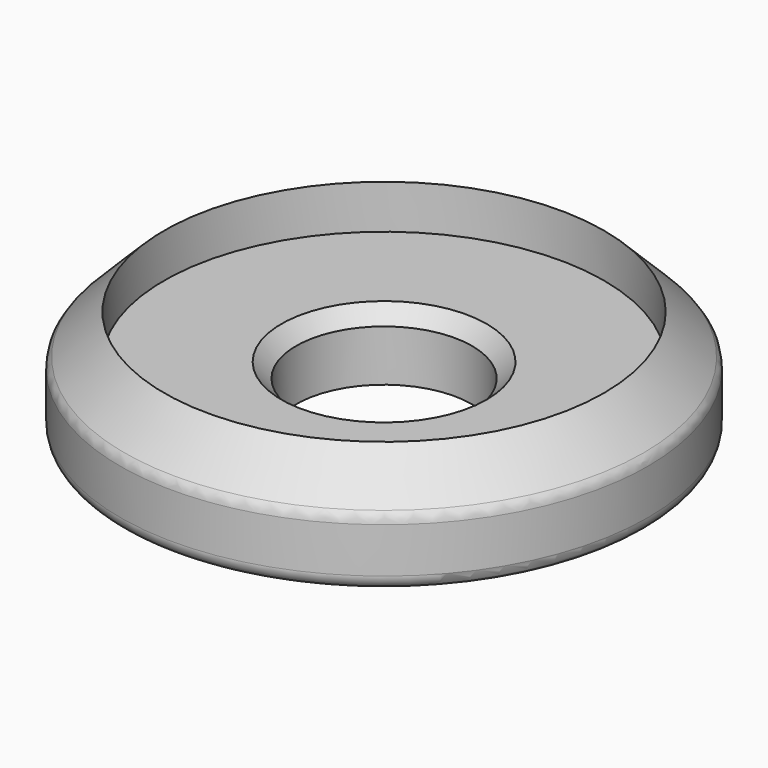
from build123d import *

# Parameters (mm, degrees)
F0_R     = 18
F1_DEPTH = 9.5
F2_R     = 15
F3_DEPTH = 5
F4_R     = 6
F5_DEPTH = 5
F6_SIZE  = 1
F8_R     = 1
F9_R     = 1


# Not quite as in the source:
# - a fillet or chamfer that OpenCascade refuses, or shapes differently, is made with other operations: its cross-section is extruded or revolved along the edge and cut away or added


with BuildPart() as f1:
    # F0 (on Top) → F1 (new body)
    with BuildSketch(Plane.XY):
        Circle(F0_R)
    extrude(amount=F1_DEPTH)

    # F2 (on face) → F3 (cut)
    with BuildSketch(Plane.XY.offset(9.5)):
        Circle(F2_R)
    extrude(amount=-F3_DEPTH, mode=Mode.SUBTRACT)

    # F4 (on Top) → F5 (cut)
    with BuildSketch(Plane.XY):
        Circle(F4_R)
    extrude(amount=F5_DEPTH, mode=Mode.SUBTRACT)

    # F6
    f6_edges = [f1.edges().sort_by_distance(p)[0] for p in [
        (-6, 0, 4.5),
    ]]
    chamfer(f6_edges, length=F6_SIZE)

    # F7: chamfer of 5 on 1 edges, made by hand

    # F7_s1 → F7_t2 (revolve, cut)
    with BuildSketch(Plane.XZ):
        Polygon((18, 4.5), (13, 9.5), (18, 9.5), align=None)
    revolve(axis=Axis((0, 0, 9.5), (0, 0, 1)), mode=Mode.SUBTRACT)

    # F8
    f8_edges = [f1.edges().sort_by_distance(p)[0] for p in [
        (-18, 0, 4.5),
    ]]
    fillet(f8_edges, radius=F8_R)

    # F9
    f9_edges = [f1.edges().sort_by_distance(p)[0] for p in [
        (-18, 0, 0),
    ]]
    fillet(f9_edges, radius=F9_R)


solid = f1.part
